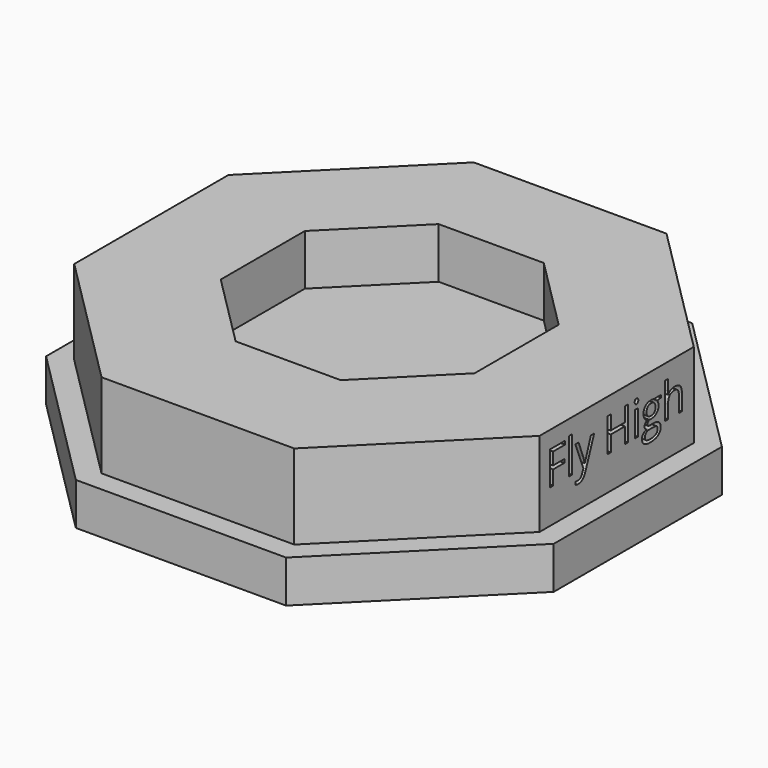
from build123d import *

# Parameters (mm, degrees)
F1_DEPTH     = 6.35
F3_DEPTH     = 12.7
F4_TEXT_SIZE = 7.0555555556
F5_DEPTH     = 6.35
F7_DEPTH     = 7.62


# Not quite as in the source:
# - Text() gives the source's letters only with a copy of the font that has no kerning and outlines rounded to 1/6400 em; it was checked with that copy


with BuildPart() as f1:
    # F0 (on Top) → F1 (new body)
    with BuildSketch(Plane.XY):
        Polygon((38.1, -15.7815367264), (38.1, 15.7815367264), (15.7815367264, 38.1), (-15.7815367264, 38.1), (-38.1, 15.7815367264), (-38.1, -15.7815367264), (-15.7815367264, -38.1), (15.7815367264, -38.1), align=None)
    extrude(amount=F1_DEPTH)

    # F2 (on face) → F3 (join)
    with BuildSketch(Plane.XY.offset(6.35)):
        Polygon((-34.925, 14.4664086659), (-34.925, -14.4664086659), (-14.4664086659, -34.925), (14.4664086659, -34.925), (34.925, -14.4664086659), (34.925, 14.4664086659), (14.4664086659, 34.925), (-14.4664086659, 34.925), align=None)
    extrude(amount=F3_DEPTH)

    # F4 (on face) → F5 (cut)
    with BuildSketch(Plane.YZ.offset(34.925)):
        with Locations((-13.1964086659, 11.43)):
            Text('Fly High', F4_TEXT_SIZE, font='Open Sans', text_align=(TextAlign.LEFT, TextAlign.BOTTOM))
    extrude(amount=-F5_DEPTH, mode=Mode.SUBTRACT)

    # F6 (on face) → F7 (cut)
    with BuildSketch(Plane.XY.offset(19.05)):
        Polygon((7.8907683632, 20.1194116146), (-7.8907683632, 20.1194116146), (-19.05, 8.9601799779), (-19.05, -6.8213567486), (-7.8907683632, -17.9805883854), (7.8907683632, -17.9805883854), (19.05, -6.8213567486), (19.05, 8.9601799779), align=None)
    extrude(amount=-F7_DEPTH, mode=Mode.SUBTRACT)


solid = f1.part
